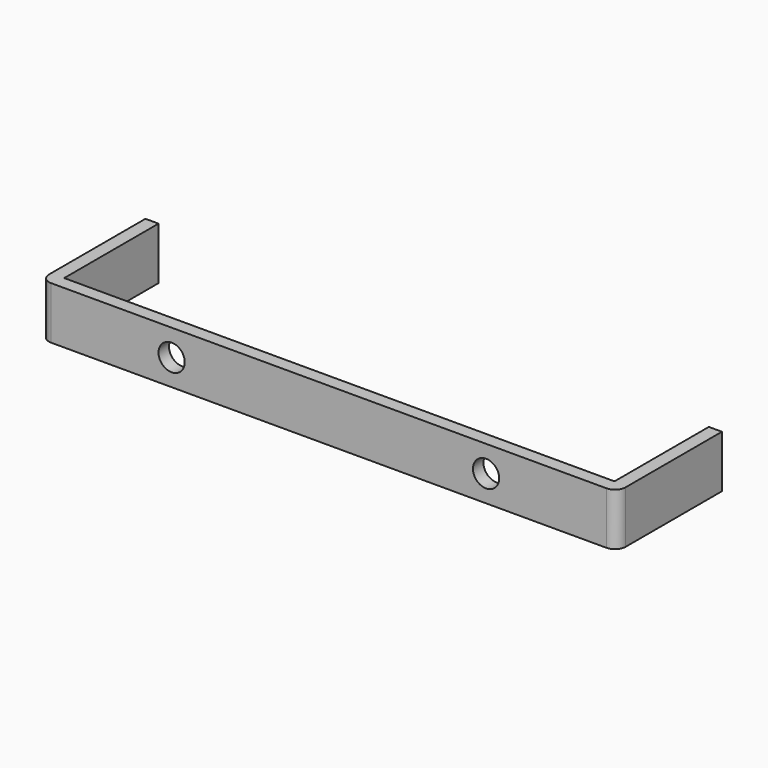
from build123d import *

# Parameters (mm, degrees)
F0_W     = 110
F0_H     = 10
F0_R     = 2.5
F1_DEPTH = 25
F2_T     = -2.5
F3_R     = 2


# Not quite as in the source:
# - a feature names something its author has since deleted; it is built from what else it names


with BuildPart() as f1:
    # F0 (on Front) → F1 (new body)
    with BuildSketch(Plane.XZ):
        Rectangle(F0_W, F0_H)
        with Locations((-30, 0)):
            Circle(F0_R, mode=Mode.SUBTRACT)
        with Locations((30, 0)):
            Circle(F0_R, mode=Mode.SUBTRACT)
    extrude(amount=-F1_DEPTH)

    # F2
    f2_openings = [f1.faces().sort_by_distance(p)[0] for p in [
        (0, 12.5, -5),
        (0, 25, 0),
        (0, 12.5, 5),
        (-32.5, 12.5, 0),
        (27.5, 12.5, 0),
    ]]
    offset(amount=F2_T, openings=f2_openings)

    # F3
    f3_edges = [f1.edges().sort_by_distance(p)[0] for p in [
        (-55, 0, 0),
        (55, 0, 0),
    ]]
    fillet(f3_edges, radius=F3_R)


solid = f1.part
